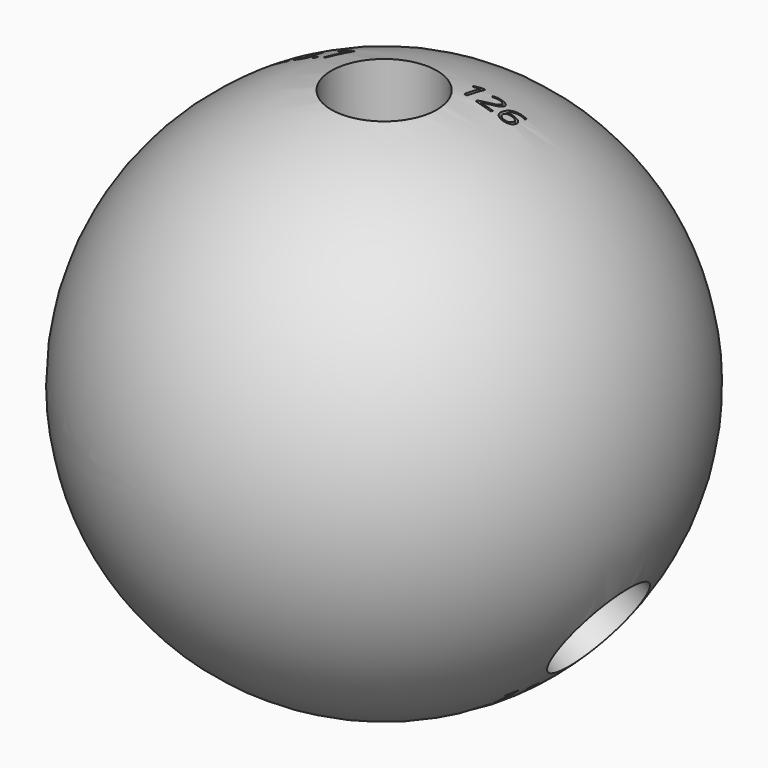
from build123d import *

# Parameters (mm, degrees)
F4_R           = 3.175
F5_DEPTH       = 25.4
F6_ANGLE       = 124
F7_ANGLE       = 112.3
F9_TEXT_SIZE   = 2.0620603916
F9_TEXT_SIZE_2 = 1.9661503352
F10_DEPTH      = 6.35
F12_TEXT_SIZE  = 2.3530398418
F13_DEPTH      = 4.572


# Not quite as in the source:
# - Text() gives the source's letters only with a copy of the font that has no kerning and outlines rounded to 1/6400 em; it was checked with that copy


with BuildPart() as f1:
    # F0 (on Top) → F1 (revolve)
    with BuildSketch(Plane.XY):
        with BuildLine():
            Line((0, -15.875), (0, 15.875))
            ThreePointArc((0, 15.875), (-15.875, 0), (0, -15.875))
        make_face()
    revolve(axis=Axis((0, 0, 0), (0, -1, 0)))

    # F9 (on offset) → F10 (cut)
    with BuildSketch(Plane.XY.offset(17.5006)):
        with Locations((-9.3983374536, 1.7085610889)):
            Text('123.7', F9_TEXT_SIZE, font='Open Sans', text_align=(TextAlign.LEFT, TextAlign.BOTTOM))
        with Locations((2.4859821424, 2.2442890331)):
            Text('126', F9_TEXT_SIZE_2, font='Open Sans', text_align=(TextAlign.LEFT, TextAlign.BOTTOM))
    extrude(amount=-F10_DEPTH, mode=Mode.SUBTRACT)

    # F12 (on offset) → F13 (cut)
    with BuildSketch(Plane(origin=(15.5404751051, 0, -10.4821828141), x_dir=(0, 1, 0), z_dir=(0.8290375726, 0, -0.5591929035))):
        with Locations((-3.5960301757, -5.594022572)):
            Text('110.3', F12_TEXT_SIZE, font='Open Sans', text_align=(TextAlign.LEFT, TextAlign.BOTTOM))
    extrude(amount=-F13_DEPTH, mode=Mode.SUBTRACT)


with BuildPart() as f5:
    # F4 (on offset) → F5 (new body)
    with BuildSketch(Plane.XY.offset(6.35)):
        Circle(F4_R)
    extrude(amount=F5_DEPTH)


with BuildPart() as f6_1:
    # F6: copy of F5
    add(f5.part.rotate(Axis((0, 19.1242676228, 0), (0, 1, 0)), F6_ANGLE))


with BuildPart() as f7_1:
    # F7: copy of F6_1
    add(f6_1.part.rotate(Axis((0, 19.1242676228, 0), (0, 1, 0)), F7_ANGLE))


with BuildPart() as f1_1:
    add(f1.part)

    # F14: cut F5, F7_1, F6_1
    add(f5.part, mode=Mode.SUBTRACT)
    add(f7_1.part, mode=Mode.SUBTRACT)
    add(f6_1.part, mode=Mode.SUBTRACT)


solid = f1_1.part
